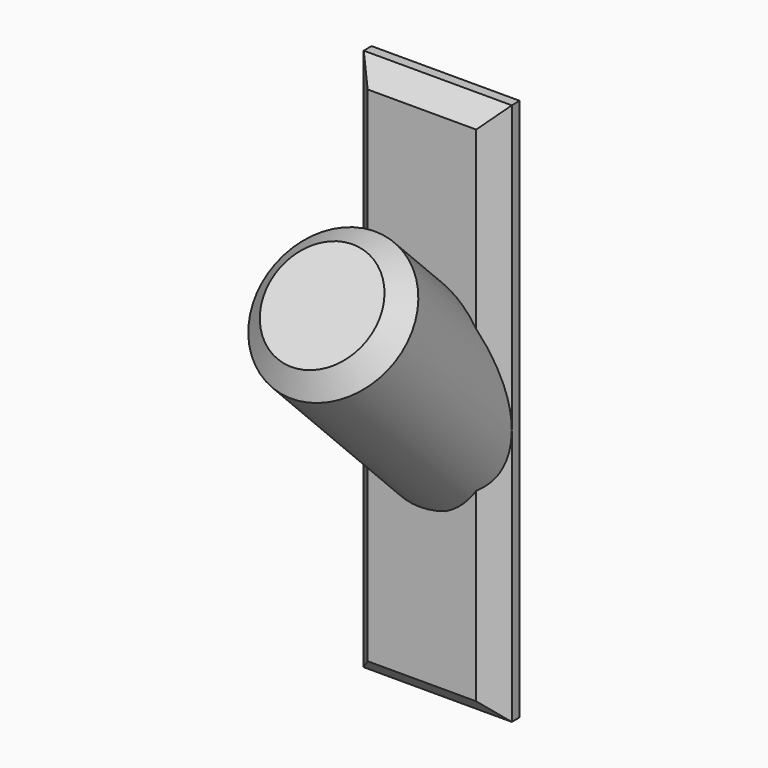
from build123d import *

# Parameters (mm, degrees)
F0_W          = 15
F0_H          = 55
F1_DEPTH      = 3
F4_R          = 7.5
F5_DEPTH      = 20
F5_DEPTH_BACK = 5
F6_T1_DEPTH   = 25.2867319519
F6_T6_DEPTH   = 32.1433659759
F6_S7_R       = 7.5
F6_T8_DEPTH   = 18
F6_T14_DEPTH  = 32.1433659759
F6_S15_R      = 7.5
F6_T16_DEPTH  = 18
F6_T20_DEPTH  = 33.1433659759
F6_S21_R      = 7.5
F6_T22_DEPTH  = 18
F6_T26_DEPTH  = 33.1433659759
F6_S27_R      = 7.5
F6_T28_DEPTH  = 18
F7_DEPTH      = 25


# Not quite as in the source:
# - a fillet or chamfer that OpenCascade refuses, or shapes differently, is made with other operations: its cross-section is extruded or revolved along the edge and cut away or added


with BuildPart() as f1:
    # F0 (on Front) → F1 (new body)
    with BuildSketch(Plane.XZ):
        with Locations((0, 2.5)):
            Rectangle(F0_W, F0_H)
    extrude(amount=F1_DEPTH)

    # F4 (on face) → F5 (join, two sides)
    with BuildSketch(Plane(origin=(0, -1.5, 1.5), x_dir=(1, 0, 0), z_dir=(0, -0.7071067812, 0.7071067812))) as f5_sk:
        Circle(F4_R)
    extrude(amount=F5_DEPTH)
    extrude(f5_sk.sketch, amount=-F5_DEPTH_BACK)

    # F6: chamfer of 2 on 7 edges, made by hand

    # F6_s2 → F6_t1 (cut)
    with BuildSketch(Plane.YZ.offset(-12.6433659759)):
        Polygon((-1, 30), (-3, 28), (-3, 30), align=None)
        Polygon((-3, -23), (-1, -25), (-3, -25), align=None)
    extrude(amount=F6_T1_DEPTH, mode=Mode.SUBTRACT)


with BuildPart() as f6_tool4:
    # F6_s5 → F6_t6 (new body)
    with BuildSketch(Plane.XY.offset(35.1433659759)):
        Polygon((-5.5, -3), (-7.5, -1), (-7.5, -3), align=None)
    extrude(amount=-F6_T6_DEPTH)

    # F6_s7 → F6_t8 (cut, symmetric)
    with BuildSketch(Plane(origin=(0, -10.5358910397, 10.5358910397), x_dir=(1, 0, 0), z_dir=(0, 0.7071067812, -0.7071067812))):
        Circle(F6_S7_R)
    extrude(amount=F6_T8_DEPTH, both=True, mode=Mode.SUBTRACT)


with BuildPart() as f1_1:
    add(f1.part)

    # F6_t3: cut F6_tool4
    add(f6_tool4.part, mode=Mode.SUBTRACT)

    # F6_s9 → F6_t10 (revolve, cut)
    with BuildSketch(Plane(origin=(0, 0, 0), x_dir=(1, 0, 0), z_dir=(0, -0.7071067812, -0.7071067812))):
        Polygon((7.5, 20.1213203436), (5.5, 22.1213203436), (7.5, 22.1213203436), align=None)
    revolve(axis=Axis((0, -15.6421356237, 15.6421356237), (0, -0.7071067812, 0.7071067812)), mode=Mode.SUBTRACT)


with BuildPart() as f6_tool12:
    # F6_s13 → F6_t14 (new body)
    with BuildSketch(Plane.XY.offset(3)):
        Polygon((5.5, -3), (7.5, -1), (7.5, -3), align=None)
    extrude(amount=F6_T14_DEPTH)

    # F6_s15 → F6_t16 (cut, symmetric)
    with BuildSketch(Plane(origin=(0, -10.5358910397, 10.5358910397), x_dir=(1, 0, 0), z_dir=(0, 0.7071067812, -0.7071067812))):
        Circle(F6_S15_R)
    extrude(amount=F6_T16_DEPTH, both=True, mode=Mode.SUBTRACT)


with BuildPart() as f1_2:
    add(f1_1.part)

    # F6_t11: cut F6_tool12
    add(f6_tool12.part, mode=Mode.SUBTRACT)


with BuildPart() as f6_tool18:
    # F6_s19 → F6_t20 (new body)
    with BuildSketch(Plane.XY.offset(-30.1433659759)):
        Polygon((5.5, -3), (7.5, -1), (7.5, -3), align=None)
    extrude(amount=F6_T20_DEPTH)

    # F6_s21 → F6_t22 (cut, symmetric)
    with BuildSketch(Plane(origin=(0, 5.7982756057, -5.7982756057), x_dir=(1, 0, 0), z_dir=(0, 0.7071067812, -0.7071067812))):
        Circle(F6_S21_R)
    extrude(amount=F6_T22_DEPTH, both=True, mode=Mode.SUBTRACT)


with BuildPart() as f1_3:
    add(f1_2.part)

    # F6_t17: cut F6_tool18
    add(f6_tool18.part, mode=Mode.SUBTRACT)


with BuildPart() as f6_tool24:
    # F6_s25 → F6_t26 (new body)
    with BuildSketch(Plane.XY.offset(3)):
        Polygon((-5.5, -3), (-7.5, -1), (-7.5, -3), align=None)
    extrude(amount=-F6_T26_DEPTH)

    # F6_s27 → F6_t28 (cut, symmetric)
    with BuildSketch(Plane(origin=(0, 5.7982756057, -5.7982756057), x_dir=(1, 0, 0), z_dir=(0, 0.7071067812, -0.7071067812))):
        Circle(F6_S27_R)
    extrude(amount=F6_T28_DEPTH, both=True, mode=Mode.SUBTRACT)


with BuildPart() as f1_4:
    add(f1_3.part)

    # F6_t23: cut F6_tool24
    add(f6_tool24.part, mode=Mode.SUBTRACT)

    # F0 (on Front) → F7 (cut)
    with BuildSketch(Plane.XZ):
        with Locations((0, 2.5)):
            Rectangle(F0_W, F0_H)
    extrude(amount=-F7_DEPTH, mode=Mode.SUBTRACT)


solid = f1_4.part
